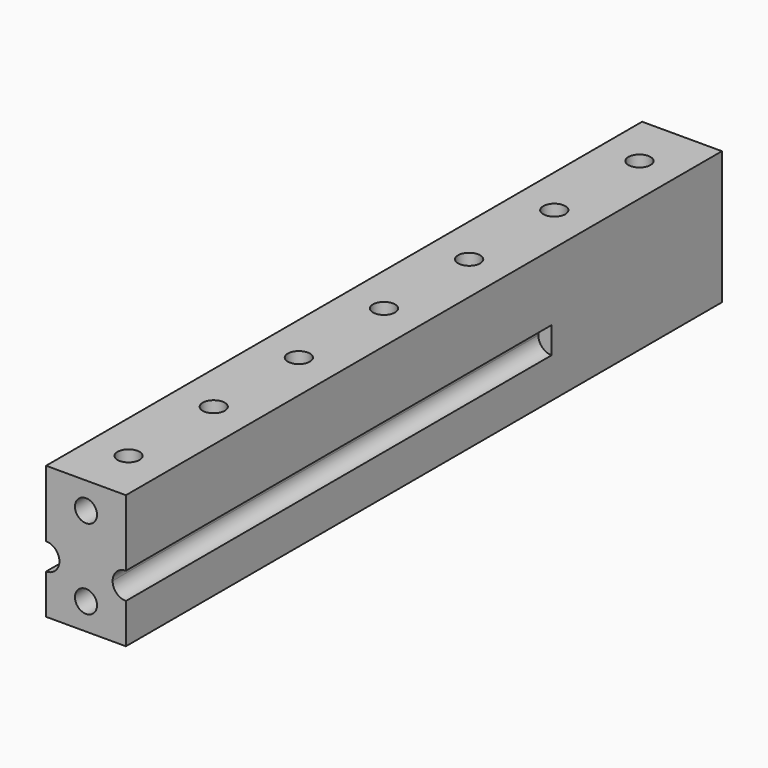
from build123d import *

# Parameters (mm, degrees)
F0_W     = 15
F0_H     = 140
F0_R     = 2.074
F1_DEPTH = 25
F3_DEPTH = 100
F4_D     = 6
F4_DEPTH = 2
F4_TIP   = 1.8025818571
F6_R     = 2.074
F7_DEPTH = 7


# Not quite as in the source:
# - a pattern or mirror of a feature is missing from the dataset's text; its kind, count and spacing are read off the source's solid


with BuildPart() as f1:
    # F0 (on Top) → F1 (new body)
    with BuildSketch(Plane.XY):
        with Locations((0, 20)):
            Rectangle(F0_W, F0_H)
        with Locations((0, -40)):
            Circle(F0_R, mode=Mode.SUBTRACT)
        with Locations((0, -20)):
            Circle(F0_R, mode=Mode.SUBTRACT)
        Circle(F0_R, mode=Mode.SUBTRACT)
        with Locations((0, 20)):
            Circle(F0_R, mode=Mode.SUBTRACT)
        with Locations((0, 40)):
            Circle(F0_R, mode=Mode.SUBTRACT)
        with Locations((0, 60)):
            Circle(F0_R, mode=Mode.SUBTRACT)
        with Locations((0, 80)):
            Circle(F0_R, mode=Mode.SUBTRACT)
    extrude(amount=F1_DEPTH)

    # F2 (on face) → F3 (cut)
    with BuildSketch(Plane.XZ.offset(50)):
        with BuildLine():
            ThreePointArc((-7.5, 7.5), (-5.732233047, 8.232233047), (-5, 10))
            ThreePointArc((-5, 10), (-5.732233047, 11.767766953), (-7.5, 12.5))
            Line((-7.5, 12.5), (-7.5, 7.5))
        make_face()
        with BuildLine():
            Line((-7.5, 7.5), (-7.5, 12.5))
            ThreePointArc((-7.5, 12.5), (-10, 10), (-7.5, 7.5))
        make_face()
    f3 = extrude(amount=-F3_DEPTH, mode=Mode.SUBTRACT)

    # F3_copies: F3 across plane
    add(f3.mirror(Plane(origin=(0, 0, 0), x_dir=(0, 0, 1), z_dir=(1, 0, 0))), mode=Mode.SUBTRACT)

    # F4
    with Locations(Plane(origin=(0, 0, 0), x_dir=(1, 0, 0), z_dir=(0, 0, -1))):
        with Locations((0, 40), (0, 20), (0, 0), (0, -20), (0, -40), (0, -60), (0, -80)):
            Hole(F4_D / 2, depth=F4_DEPTH)
            with Locations((0, 0, -(F4_DEPTH + F4_TIP / 2))):  # 118° drill point
                Cone(0, F4_D / 2, F4_TIP, mode=Mode.SUBTRACT)

    # F6 (on face) → F7 (cut)
    with BuildSketch(Plane.XZ.offset(50)):
        with Locations((0, 5)):
            Circle(F6_R)
        with Locations((0, 20)):
            Circle(F6_R)
    extrude(amount=-F7_DEPTH, mode=Mode.SUBTRACT)


solid = f1.part
